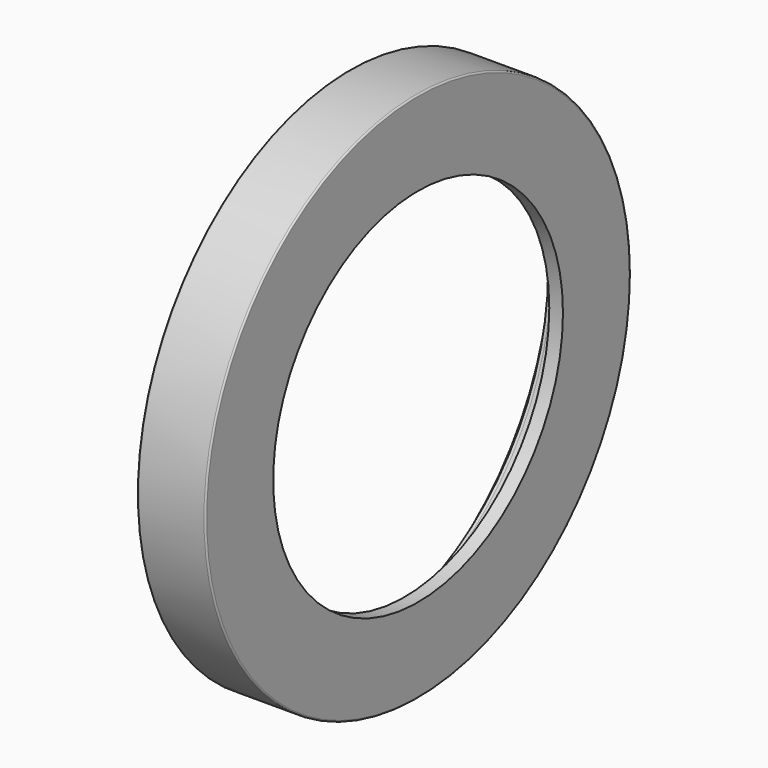
from build123d import *

# Parameters (mm, degrees)
F2_R = 0.13


# Not quite as in the source:
# - a feature names something its author has since deleted; it is built from what else it names


with BuildPart() as f1:
    # F0 (on Top) → F1 (revolve)
    with BuildSketch(Plane.XY):
        with BuildLine():
            Line((7.3, 15.1), (7.3, 22.16))
            Line((7.3, 22.16), (1.6, 22.16))
            Line((1.6, 22.16), (1.6, 20.79))
            Line((1.6, 20.79), (2.9, 20.79))
            Line((2.9, 20.79), (2.9, 19.05))
            Line((2.9, 19.05), (3.16, 19.05))
            ThreePointArc((3.16, 19.05), (5.2813203436, 18.1713203436), (6.16, 16.05))
            Line((6.16, 16.05), (6.16, 15.1))
            Line((6.16, 15.1), (7.3, 15.1))
        make_face()
    revolve(axis=Axis((7.0380799007, 0, 0), (1, 0, 0)))

    # F2
    f2_edges = [f1.edges().sort_by_distance(p)[0] for p in [
        (7.3, -22.16, 0),
        (1.6, -22.16, 0),
        (1.6, -20.79, 0),
    ]]
    fillet(f2_edges, radius=F2_R)


solid = f1.part
